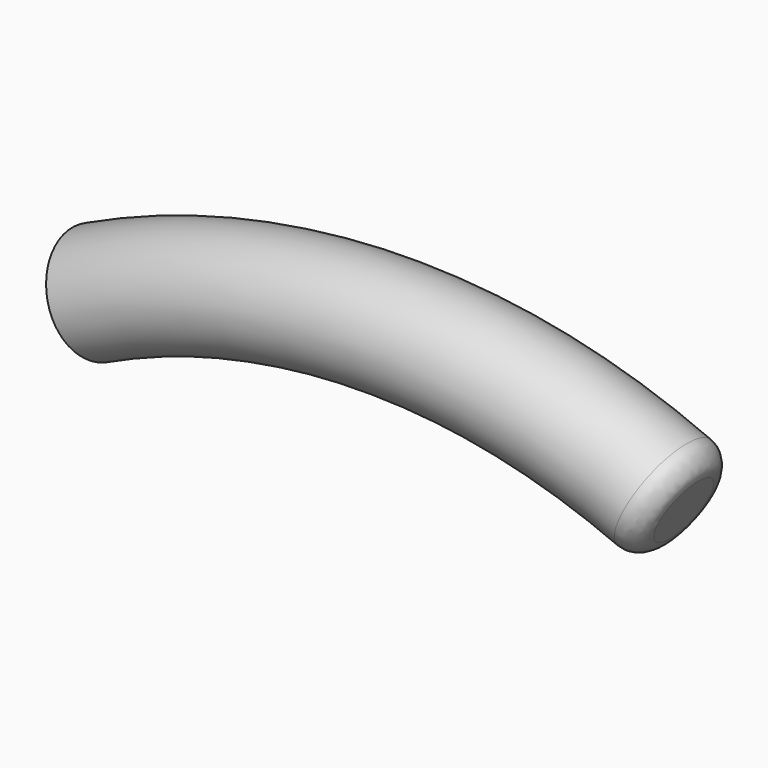
from build123d import *

# Parameters (mm, degrees)
F2_R = 12.7
F4_R = 5.08
F5_T = -2.54


with BuildPart() as f3:
    # F3: sweep along a path in F0
    with BuildLine(Plane.XZ) as f3_path:
        ThreePointArc((62.0554685593, 0), (-5.6746825576, 15.2487086239), (-73.4048336744, 0))
    # F2 (on line) → F3 (sweep)
    with BuildSketch(Plane(origin=(50.6583556933, 0, -24.0282957665), x_dir=(0, -1, 0), z_dir=(-0.9035153077, 0, 0.4285558176))):
        with Locations((0, 26.5942320649)):
            Circle(F2_R)
    sweep(path=f3_path.line)

    # F4
    f4_edges = [f3.edges().sort_by_distance(p)[0] for p in [
        (62.055469, 12.7, 0),
    ]]
    fillet(f4_edges, radius=F4_R)

    # F5
    f5_openings = [f3.faces().sort_by_distance(p)[0] for p in [
        (-73.404834, 0, 0),
    ]]
    offset(amount=F5_T, openings=f5_openings)


solid = f3.part
